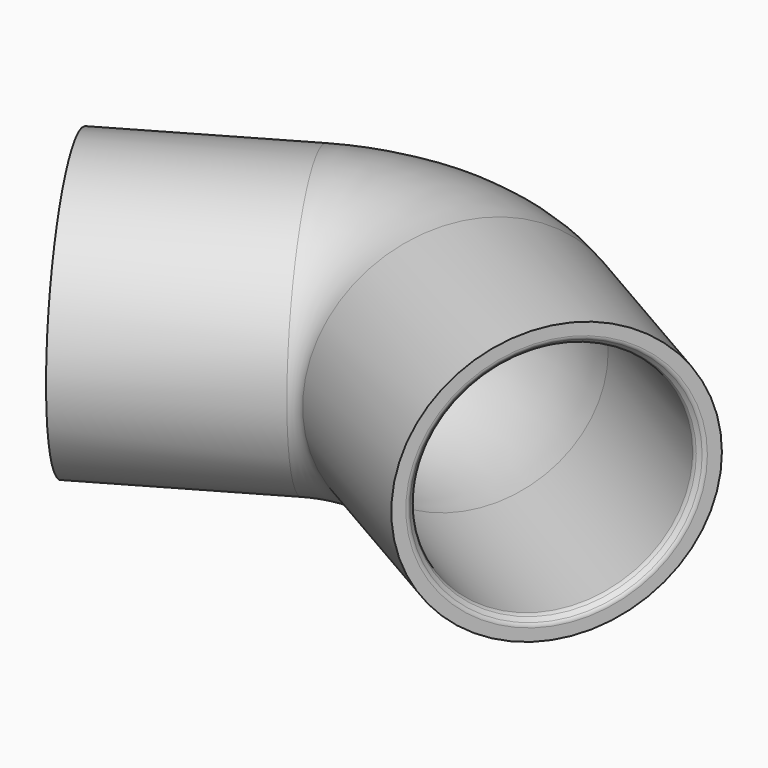
from build123d import *

# Parameters (mm, degrees)
F1_R    = 13.1633
F1_R_2  = 11.1633
F3_SIZE = 0.635
F4_R    = 0.508


with BuildPart() as f2:
    # F2: sweep along a path in F0
    with BuildLine(Plane.XY) as f2_path:
        Line((-21.9970452561, -12.7), (-6.35, -3.6661742094))
        ThreePointArc((-6.35, -3.6661742094), (0, -1.9646968374), (6.35, -3.6661742094))
        Line((6.35, -3.6661742094), (21.9970452561, -12.7))
    # F1 (on Right) → F2 (sweep)
    with BuildSketch(Plane.YZ):
        Circle(F1_R)
        Circle(F1_R_2, mode=Mode.SUBTRACT)
    sweep(path=f2_path.line)

    # F3
    f3_edges = [f2.edges().sort_by_distance(p)[0] for p in [
        (17.397744, -20.666224, 0),
        (-17.397744, -20.666224, 0),
    ]]
    chamfer(f3_edges, length=F3_SIZE)

    # F4
    f4_edges = [f2.edges().sort_by_distance(p)[0] for p in [
        (-17.080244, -21.21615, 0),
        (-16.847818, -20.348724, 0),
        (16.847818, -20.348724, 0),
        (17.080244, -21.21615, 0),
    ]]
    fillet(f4_edges, radius=F4_R)


solid = f2.part
